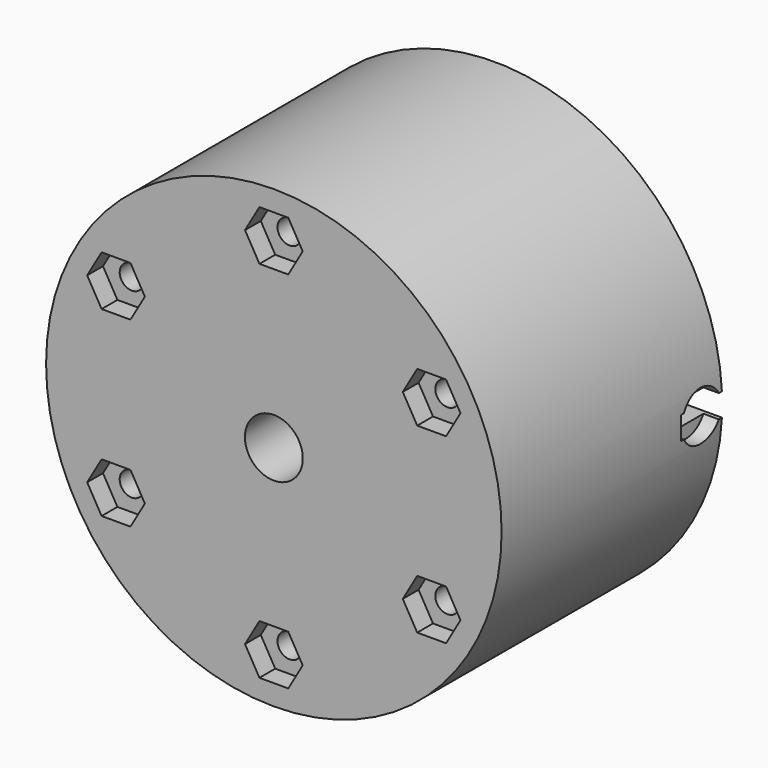
from build123d import *

# Parameters (mm, degrees)
F0_R            = 37.5
F1_DEPTH        = 45.4
F2_R            = 2
F3_DEPTH        = 45.401
F3_COPIES_COUNT = 6
F5_DEPTH        = 3.25
F5_COPIES_COUNT = 6
F7_DEPTH        = 8.4582
F8_W            = 76.2
F8_H            = 3.81
F9_DEPTH        = 8.4582
F11_R           = 4.064
F12_DEPTH       = 2.54
F13_R           = 4.7625
F14_DEPTH       = 36.9428001


# Not quite as in the source:
# - a pattern or mirror of a feature is missing from the dataset's text; its kind, count and spacing are read off the source's solid


with BuildPart() as f1:
    # F0 (on Front) → F1 (new body)
    with BuildSketch(Plane.XZ):
        Circle(F0_R)
    extrude(amount=F1_DEPTH)

    # F2 (on Front) → F3 (cut, through all)
    with BuildSketch(Plane.XZ):
        with Locations((0, 30)):
            Circle(F2_R)
    f3 = extrude(amount=F3_DEPTH, mode=Mode.SUBTRACT)

    # F3_copies: F3 ×6 about axis
    f3_copies_axis = Axis((0, 0, 0), (0, 1, 0))
    for i in range(1, F3_COPIES_COUNT):
        add(f3.rotate(f3_copies_axis, i * 360 / F3_COPIES_COUNT), mode=Mode.SUBTRACT)

    # F4 (on face) → F5 (cut)
    with BuildSketch(Plane.XZ.offset(45.4)):
        Polygon((2.3749, 34.1134474629), (-2.3749, 34.1134474629), (-4.7498, 30), (-2.3749, 25.8865525371), (2.3749, 25.8865525371), (4.7498, 30), align=None)
    f5 = extrude(amount=-F5_DEPTH, mode=Mode.SUBTRACT)

    # F5_copies: F5 ×6 about axis
    f5_copies_axis = Axis((0, 0, 0), (0, 1, 0))
    for i in range(1, F5_COPIES_COUNT):
        add(f5.rotate(f5_copies_axis, i * 360 / F5_COPIES_COUNT), mode=Mode.SUBTRACT)

    # F6 (on face) → F7 (cut)
    with BuildSketch(Plane(origin=(0, 0, 0), x_dir=(-1, 0, 0), z_dir=(0, 1, 0))):
        Polygon((-4.1574415534, -7.2009), (4.1574415534, -7.2009), (8.3148831068, 0), (4.1574415534, 7.2009), (-4.1574415534, 7.2009), (-8.3148831068, 0), align=None)
    extrude(amount=-F7_DEPTH, mode=Mode.SUBTRACT)

    # F8 (on face) → F9 (cut, through all)
    with BuildSketch(Plane(origin=(0, 0, 0), x_dir=(-1, 0, 0), z_dir=(0, 1, 0))):
        Rectangle(F8_W, F8_H)
    extrude(amount=-F9_DEPTH, mode=Mode.SUBTRACT)

    # F11 (on 3pt) → F12 (cut)
    with BuildSketch(Plane.YZ.offset(37.4515817423)):
        with Locations((-4.2291, 0)):
            Circle(F11_R)
    extrude(amount=-F12_DEPTH, mode=Mode.SUBTRACT)

    # F13 (on face) → F14 (cut, through all)
    with BuildSketch(Plane(origin=(0, -8.4582, 0), x_dir=(-1, 0, 0), z_dir=(0, 1, 0))):
        Circle(F13_R)
    extrude(amount=-F14_DEPTH, mode=Mode.SUBTRACT)


solid = f1.part
